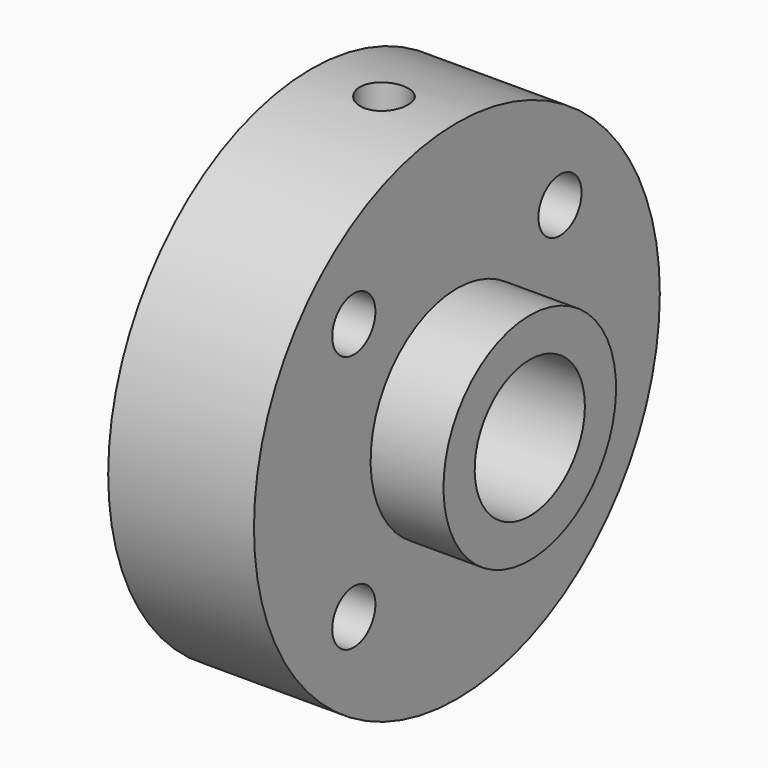
from build123d import *

# Parameters (mm, degrees)
F3_D            = 2.35
F3_COPIES_COUNT = 4
F7_D            = 2.1
F7_DEPTH        = 8.5
F7_START        = 0.0500046
F7_TIP          = 0.63090365


# Not quite as in the source:
# - a pattern or mirror of a feature is missing from the dataset's text; its kind, count and spacing are read off the source's solid


with BuildPart() as f1:
    # F0 (on Front) → F1 (revolve)
    with BuildSketch(Plane.XZ):
        Polygon((-6.35, 4.699), (-6.35, 3), (6.35, 3), (6.35, 4.699), (3.175, 4.699), (3.175, 11.049), (-3.175, 11.049), (-3.175, 4.699), align=None)
    revolve(axis=Axis((0, 0, 0), (1, 0, 0)))

    # F3 (through all)
    with Locations(Plane(origin=(-3.175, 0, 0), x_dir=(0, -1, 0), z_dir=(-1, 0, 0))):
        with Locations((5.6126600757, 5.6126600757)):
            f3 = Hole(F3_D / 2)

    # F3_copies: F3 ×4 about axis
    f3_copies_axis = Axis((0, 0, 0), (1, 0, 0))
    for i in range(1, F3_COPIES_COUNT):
        add(f3.rotate(f3_copies_axis, i * 360 / F3_COPIES_COUNT), mode=Mode.SUBTRACT)

    # F7
    # its depths count from where the whole tool has entered the part; down to there all is cleared
    with Locations(Plane.XY.offset(11.049).offset(-F7_START)):
        with Locations((0, 0)):
            Hole(F7_D / 2, depth=F7_DEPTH)
            with Locations((0, 0, -(F7_DEPTH + F7_TIP / 2))):  # 118° drill point
                Cone(0, F7_D / 2, F7_TIP, mode=Mode.SUBTRACT)


solid = f1.part
